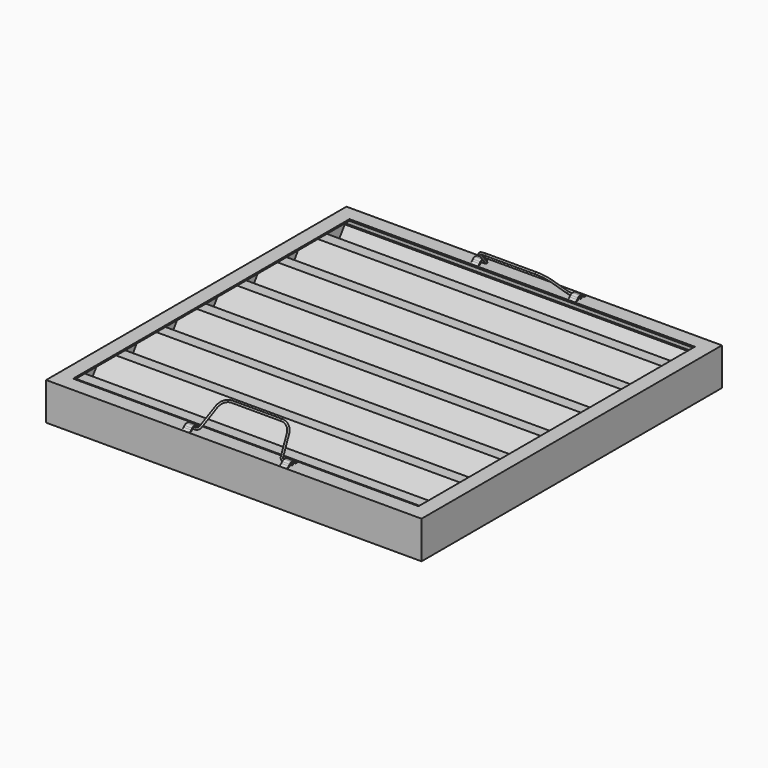
from build123d import *

# Parameters (mm, degrees)
F4_DEPTH = 496
F7_DEPTH = 10
F9_R     = 5
F14_R    = 1.25


with BuildPart() as f2:
    # F2: sweep along a path in F1
    with BuildLine(Plane.XY) as f2_path:
        Line((-250, 250), (250, 250))
        Line((250, 250), (250, -250))
        Line((250, -250), (-250, -250))
        Line((-250, -250), (-250, 250))
    # F0 (on Right) → F2 (sweep)
    with BuildSketch(Plane.YZ):
        Polygon((250, 10), (230, 10), (230, 8), (248, 8), (248, -38), (230, -38), (230, -40), (250, -40), align=None)
    sweep(path=f2_path.line, transition=Transition.RIGHT)

    # F3 (on face) → F4 (join, through all)
    with BuildSketch(Plane.YZ.offset(-248)):
        Polygon((-225.4937738537, 8), (-246.5, -22), (-244.0584508225, -22), (-224.4526397526, 6), (-211.5349079548, 6), (-191.9290968849, -22), (-189.4875477074, -22), (-210.4937738537, 8), align=None)
        Polygon((-210.2774245412, -8), (-212.7189737187, -8), (-191.7127475724, -38), (-176.7127475724, -38), (-155.7065214261, -8), (-158.1480706037, -8), (-177.7538816735, -36), (-190.6716134713, -36), align=None)
        Polygon((-124.5633975724, -38), (-109.5633975724, -38), (-88.5571714261, -8), (-90.9987206037, -8), (-110.6045316735, -36), (-123.5222634713, -36), (-143.1280745412, -8), (-145.5696237187, -8), align=None)
        Polygon((-157.3032897526, 6), (-144.3855579548, 6), (-124.7797468849, -22), (-122.3381977074, -22), (-143.3444238537, 8), (-158.3444238537, 8), (-179.35065, -22), (-176.9091008225, -22), align=None)
        Polygon((-57.4140475724, -38), (-42.4140475724, -38), (-21.4078214261, -8), (-23.8493706037, -8), (-43.4551816735, -36), (-56.3729134713, -36), (-75.9787245412, -8), (-78.4202737187, -8), align=None)
        Polygon((-90.1539397526, 6), (-77.2362079548, 6), (-57.6303968849, -22), (-55.1888477074, -22), (-76.1950738537, 8), (-91.1950738537, 8), (-112.2013, -22), (-109.7597508225, -22), align=None)
        Polygon((9.7353024276, -38), (24.7353024276, -38), (45.7415285739, -8), (43.2999793963, -8), (23.6941683265, -36), (10.7764365287, -36), (-8.8293745412, -8), (-11.2709237187, -8), align=None)
        Polygon((-23.0045897526, 6), (-10.0868579548, 6), (9.5189531151, -22), (11.9605022926, -22), (-9.0457238537, 8), (-24.0457238537, 8), (-45.05195, -22), (-42.6104008225, -22), align=None)
        Polygon((76.8846524276, -38), (91.8846524276, -38), (112.8908785739, -8), (110.4493293963, -8), (90.8435183265, -36), (77.9257865287, -36), (58.3199754588, -8), (55.8784262813, -8), align=None)
        Polygon((44.1447602474, 6), (57.0624920452, 6), (76.6683031151, -22), (79.1098522926, -22), (58.1036261463, 8), (43.1036261463, 8), (22.0974, -22), (24.5389491775, -22), align=None)
        Polygon((144.0340024276, -38), (159.0340024276, -38), (180.0402285739, -8), (177.5986793963, -8), (157.9928683265, -36), (145.0751365287, -36), (125.4693254588, -8), (123.0277762813, -8), align=None)
        Polygon((111.2941102474, 6), (124.2118420452, 6), (143.8176531151, -22), (146.2592022926, -22), (125.2529761463, 8), (110.2529761463, 8), (89.24675, -22), (91.6882991775, -22), align=None)
        Polygon((211.1833524276, -38), (226.1833524276, -38), (247.1895785739, -8), (244.7480293963, -8), (225.1422183265, -36), (212.2244865287, -36), (192.6186754588, -8), (190.1771262813, -8), align=None)
        Polygon((178.4434602474, 6), (191.3611920452, 6), (210.9670031151, -22), (213.4085522926, -22), (192.4023261463, 8), (177.4023261463, 8), (156.3961, -22), (158.8376491775, -22), align=None)
    extrude(amount=F4_DEPTH)

    # F6 (on offset) → F7 (join)
    with BuildSketch(Plane.YZ.offset(60)):
        Polygon((245.3786796564, 10), (247.5, 10), (243, 14.5), (237, 14.5), (232.5, 10), (234.6213203436, 10), (237.6213203436, 13), (242.3786796564, 13), align=None)
        Polygon((-234.6213203436, 10), (-232.5, 10), (-237, 14.5), (-243, 14.5), (-247.5, 10), (-245.3786796564, 10), (-242.3786796564, 13), (-237.6213203436, 13), align=None)
    extrude(amount=F7_DEPTH)

    # F8: F2 across plane


with BuildPart() as f2_1:
    add(f2.part)
    add(f2.part.mirror(Plane.YZ))

    # F9
    f9_edges = [f2_1.edges().sort_by_distance(p)[0] for p in [
        (-65, 247.5, 10),
        (-65, 243, 14.5),
        (-65, 237, 14.5),
        (-65, 232.5, 10),
        (-65, 237.62132, 13),
        (-65, 242.37868, 13),
        (65, 247.5, 10),
        (65, 243, 14.5),
        (65, 237, 14.5),
        (65, 232.5, 10),
        (65, 237.62132, 13),
        (65, 242.37868, 13),
        (-65, -232.5, 10),
        (-65, -237, 14.5),
        (-65, -243, 14.5),
        (-65, -247.5, 10),
        (-65, -242.37868, 13),
        (-65, -237.62132, 13),
        (65, -232.5, 10),
        (65, -237.62132, 13),
        (65, -237, 14.5),
        (65, -242.37868, 13),
        (65, -243, 14.5),
        (65, -247.5, 10),
    ]]
    fillet(f9_edges, radius=F9_R)


with BuildPart() as f15:
    # F15: sweep along a path in F13
    with BuildLine(Plane(origin=(0, 125.625, 125.625), x_dir=(1, 0, 0), z_dir=(0, -0.7071067812, -0.7071067812))) as f15_path:
        Line((70, -161.7315501512), (58.903882032, -161.7315501512))
        ThreePointArc((58.903882032, -161.7315501512), (55.826820985, -160.6725773412), (54.0531695313, -157.9442282763))
        Line((54.0531695313, -157.9442282763), (47.8404914061, -133.0935157756))
        ThreePointArc((47.8404914061, -133.0935157756), (42.519537045, -124.9084685809), (33.2883539039, -121.7315501512))
        Line((33.2883539039, -121.7315501512), (-33.2883539039, -121.7315501512))
        ThreePointArc((-33.2883539039, -121.7315501512), (-42.519537045, -124.9084685809), (-47.8404914061, -133.0935157756))
        Line((-47.8404914061, -133.0935157756), (-54.0531695313, -157.9442282763))
        ThreePointArc((-54.0531695313, -157.9442282763), (-55.826820985, -160.6725773412), (-58.903882032, -161.7315501512))
        Line((-58.903882032, -161.7315501512), (-70, -161.7315501512))
    # F14 (on Right) → F15 (sweep)
    with BuildSketch(Plane.YZ):
        with Locations((211.7022045962, 39.5477954038)):
            Circle(F14_R)
    sweep(path=f15_path.line)


with BuildPart() as f16_1:
    # F16: instance of F15
    add(f15.part.mirror(Plane.XZ))


solid = Compound([f2_1.part, f15.part, f16_1.part])
